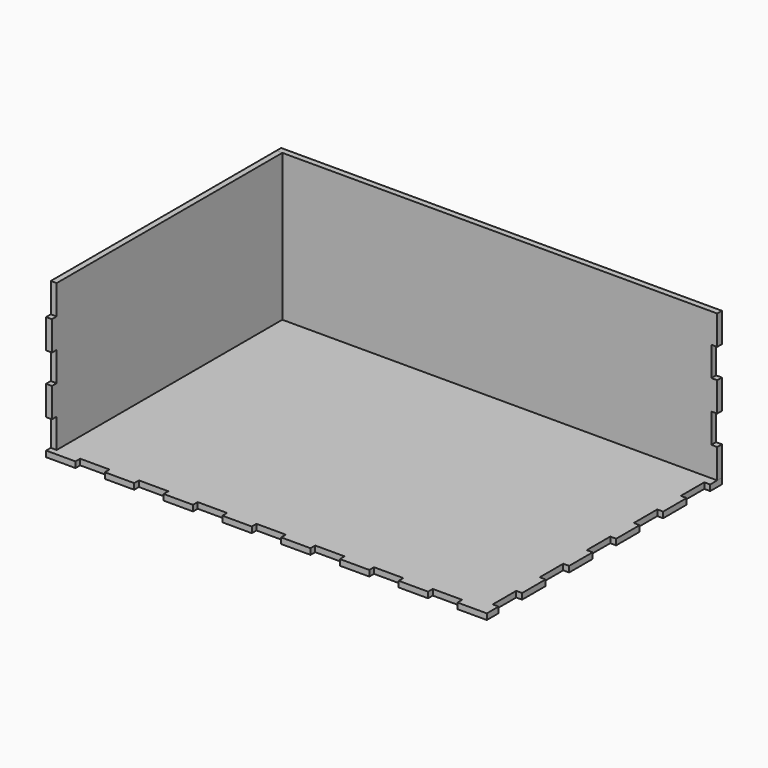
from build123d import *

# Parameters (mm, degrees)
F1_DEPTH  = 4
F2_W      = 20
F2_H      = 4
F3_DEPTH  = 4
F4_W      = 20
F4_H      = 4
F5_DEPTH  = 100
F7_W      = 4
F7_H      = 20
F8_DEPTH  = 4
F9_W      = 4
F9_H      = 10
F9_H_2    = 20
F10_DEPTH = 100
F12_W     = 4
F12_H     = 20
F13_DEPTH = 4
F14_W     = 4
F14_H     = 20
F15_DEPTH = 4


with BuildPart() as f1:
    # F0 (on Top) → F1 (new body)
    with BuildSketch(Plane.XY):
        Polygon((150, 90), (150, 100), (130, 100), (130, 96), (120, 96), (110, 96), (110, 100), (90, 100), (90, 96), (80, 96), (70, 96), (70, 100), (50, 100), (50, 96), (40, 96), (30, 96), (30, 100), (10, 100), (10, 96), (0, 96), (-10, 96), (-10, 100), (-30, 100), (-30, 96), (-40, 96), (-50, 96), (-50, 100), (-70, 100), (-70, 96), (-80, 96), (-90, 96), (-90, 100), (-110, 100), (-110, 96), (-120, 96), (-130, 96), (-130, 100), (-150, 100), (-150, 90), (-146, 90), (-146, 80), (-146, 70), (-150, 70), (-150, 50), (-146, 50), (-146, 40), (-146, 30), (-150, 30), (-150, 10), (-146, 10), (-146, 0), (-146, -10), (-150, -10), (-150, -30), (-146, -30), (-146, -40), (-146, -50), (-150, -50), (-150, -70), (-146, -70), (-146, -80), (-146, -90), (-150, -90), (-150, -100), (-130, -100), (-130, -96), (-120, -96), (-110, -96), (-110, -100), (-90, -100), (-90, -96), (-80, -96), (-70, -96), (-70, -100), (-50, -100), (-50, -96), (-40, -96), (-30, -96), (-30, -100), (-10, -100), (-10, -96), (0, -96), (10, -96), (10, -100), (30, -100), (30, -96), (40, -96), (50, -96), (50, -100), (70, -100), (70, -96), (80, -96), (90, -96), (90, -100), (110, -100), (110, -96), (120, -96), (130, -96), (130, -100), (150, -100), (150, -90), (146, -90), (146, -80), (146, -70), (150, -70), (150, -50), (146, -50), (146, -40), (146, -30), (150, -30), (150, -10), (146, -10), (146, 0), (146, 10), (150, 10), (150, 30), (146, 30), (146, 40), (146, 50), (150, 50), (150, 70), (146, 70), (146, 80), (146, 90), align=None)
    extrude(amount=F1_DEPTH)


with BuildPart() as f3:
    # F2 (on face) → F3 (new body, through all)
    with BuildSketch(Plane.XY.offset(4)):
        with Locations((-120, 98)):
            Rectangle(F2_W, F2_H)
    extrude(amount=-F3_DEPTH)



with BuildPart() as f3b:
    # F2 (on face) → F3, piece 2 (new body, through all)
    with BuildSketch(Plane.XY.offset(4)):
        with Locations((120, 98)):
            Rectangle(F2_W, F2_H)
    extrude(amount=-F3_DEPTH)


with BuildPart() as f3c:
    # F2 (on face) → F3, piece 3 (new body, through all)
    with BuildSketch(Plane.XY.offset(4)):
        with Locations((80, 98)):
            Rectangle(F2_W, F2_H)
    extrude(amount=-F3_DEPTH)


with BuildPart() as f3d:
    # F2 (on face) → F3, piece 4 (new body, through all)
    with BuildSketch(Plane.XY.offset(4)):
        with Locations((40, 98)):
            Rectangle(F2_W, F2_H)
    extrude(amount=-F3_DEPTH)


with BuildPart() as f3e:
    # F2 (on face) → F3, piece 5 (new body, through all)
    with BuildSketch(Plane.XY.offset(4)):
        with Locations((0, 98)):
            Rectangle(F2_W, F2_H)
    extrude(amount=-F3_DEPTH)


with BuildPart() as f3f:
    # F2 (on face) → F3, piece 6 (new body, through all)
    with BuildSketch(Plane.XY.offset(4)):
        with Locations((-40, 98)):
            Rectangle(F2_W, F2_H)
    extrude(amount=-F3_DEPTH)


with BuildPart() as f3g:
    # F2 (on face) → F3, piece 7 (new body, through all)
    with BuildSketch(Plane.XY.offset(4)):
        with Locations((-80, 98)):
            Rectangle(F2_W, F2_H)
    extrude(amount=-F3_DEPTH)


with BuildPart() as f3_1:
    add(f3.part)

    add(f3b.part)  # F5 merges F3b

    add(f3c.part)  # F5 merges F3c

    add(f3d.part)  # F5 merges F3d

    add(f3e.part)  # F5 merges F3e

    add(f3f.part)  # F5 merges F3f

    add(f3g.part)  # F5 merges F3g
    # F4 (on face) → F5 (join)
    with BuildSketch(Plane.XY.offset(4)):
        with Locations((140, 98)):
            Rectangle(F4_W, F4_H)
        with Locations((120, 98)):
            Rectangle(F4_W, F4_H)
        with Locations((100, 98)):
            Rectangle(F4_W, F4_H)
        with Locations((80, 98)):
            Rectangle(F4_W, F4_H)
        with Locations((60, 98)):
            Rectangle(F4_W, F4_H)
        with Locations((40, 98)):
            Rectangle(F4_W, F4_H)
        with Locations((20, 98)):
            Rectangle(F4_W, F4_H)
        with Locations((0, 98)):
            Rectangle(F4_W, F4_H)
        with Locations((-20, 98)):
            Rectangle(F4_W, F4_H)
        with Locations((-40, 98)):
            Rectangle(F4_W, F4_H)
        with Locations((-60, 98)):
            Rectangle(F4_W, F4_H)
        with Locations((-80, 98)):
            Rectangle(F4_W, F4_H)
        with Locations((-100, 98)):
            Rectangle(F4_W, F4_H)
        with Locations((-120, 98)):
            Rectangle(F4_W, F4_H)
        with Locations((-140, 98)):
            Rectangle(F4_W, F4_H)
    extrude(amount=F5_DEPTH)

    # F6: union 

    # F14 (on face) → F15 (cut, through all)
    with BuildSketch(Plane(origin=(0, 100, 0), x_dir=(-1, 0, 0), z_dir=(0, 1, 0))):
        with Locations((-148, 74)):
            Rectangle(F14_W, F14_H)
        with Locations((-148, 34)):
            Rectangle(F14_W, F14_H)
        with Locations((148, 74)):
            Rectangle(F14_W, F14_H)
        with Locations((148, 34)):
            Rectangle(F14_W, F14_H)
    extrude(amount=-F15_DEPTH, mode=Mode.SUBTRACT)


with BuildPart() as f8:
    # F7 (on face) → F8 (new body, through all)
    with BuildSketch(Plane.XY.offset(4)):
        with Locations((-148, 80)):
            Rectangle(F7_W, F7_H)
    extrude(amount=-F8_DEPTH)



with BuildPart() as f8b:
    # F7 (on face) → F8, piece 2 (new body, through all)
    with BuildSketch(Plane.XY.offset(4)):
        with Locations((-148, 40)):
            Rectangle(F7_W, F7_H)
    extrude(amount=-F8_DEPTH)


with BuildPart() as f8c:
    # F7 (on face) → F8, piece 3 (new body, through all)
    with BuildSketch(Plane.XY.offset(4)):
        with Locations((-148, 0)):
            Rectangle(F7_W, F7_H)
    extrude(amount=-F8_DEPTH)


with BuildPart() as f8d:
    # F7 (on face) → F8, piece 4 (new body, through all)
    with BuildSketch(Plane.XY.offset(4)):
        with Locations((-148, -40)):
            Rectangle(F7_W, F7_H)
    extrude(amount=-F8_DEPTH)


with BuildPart() as f8e:
    # F7 (on face) → F8, piece 5 (new body, through all)
    with BuildSketch(Plane.XY.offset(4)):
        with Locations((-148, -80)):
            Rectangle(F7_W, F7_H)
    extrude(amount=-F8_DEPTH)


with BuildPart() as f8_1:
    add(f8.part)

    add(f8b.part)  # F10 merges F8b

    add(f8c.part)  # F10 merges F8c

    add(f8d.part)  # F10 merges F8d

    add(f8e.part)  # F10 merges F8e
    # F9 (on face) → F10 (join)
    with BuildSketch(Plane.XY.offset(4)):
        with Locations((-148, -95)):
            Rectangle(F9_W, F9_H)
        with Locations((-148, -80)):
            Rectangle(F9_W, F9_H_2)
        with Locations((-148, -60)):
            Rectangle(F9_W, F9_H_2)
        with Locations((-148, -40)):
            Rectangle(F9_W, F9_H_2)
        with Locations((-148, -20)):
            Rectangle(F9_W, F9_H_2)
        with Locations((-148, 0)):
            Rectangle(F9_W, F9_H_2)
        with Locations((-148, 20)):
            Rectangle(F9_W, F9_H_2)
        with Locations((-148, 40)):
            Rectangle(F9_W, F9_H_2)
        with Locations((-148, 60)):
            Rectangle(F9_W, F9_H_2)
        with Locations((-148, 80)):
            Rectangle(F9_W, F9_H_2)
        with Locations((-148, 95)):
            Rectangle(F9_W, F9_H)
    extrude(amount=F10_DEPTH)

    # F11: union 

    # F12 (on face) → F13 (cut, through all)
    with BuildSketch(Plane(origin=(-150, 0, 0), x_dir=(0, -1, 0), z_dir=(-1, 0, 0))):
        with Locations((-98, 14)):
            Rectangle(F12_W, F12_H)
        with Locations((-98, 54)):
            Rectangle(F12_W, F12_H)
        with Locations((-98, 94)):
            Rectangle(F12_W, F12_H)
        with Locations((98, 14)):
            Rectangle(F12_W, F12_H)
        with Locations((98, 54)):
            Rectangle(F12_W, F12_H)
        with Locations((98, 94)):
            Rectangle(F12_W, F12_H)
    extrude(amount=-F13_DEPTH, mode=Mode.SUBTRACT)


solid = Compound([f1.part, f3_1.part, f8_1.part])
